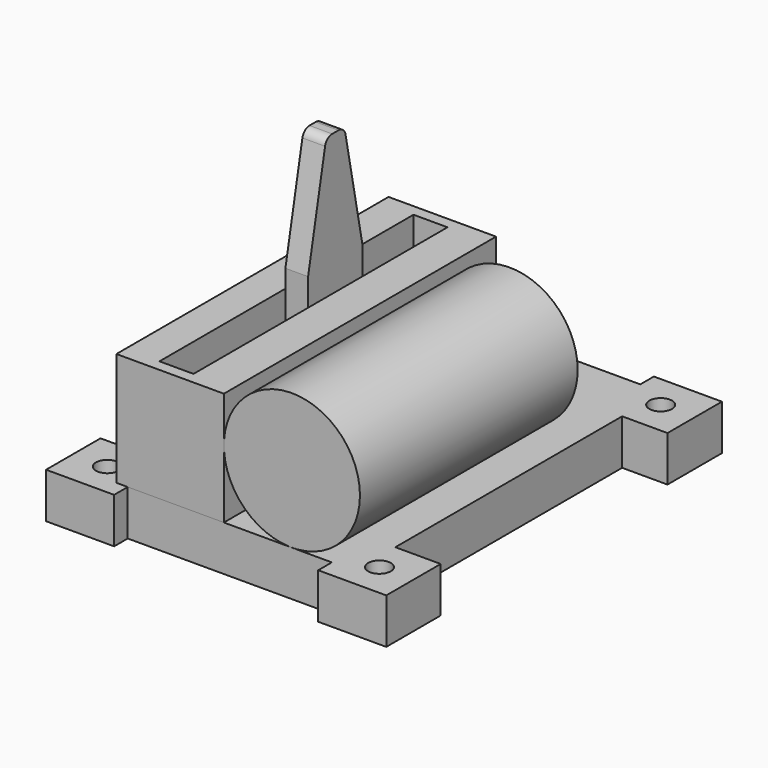
from build123d import *

# Parameters (mm, degrees)
F0_R     = 0.5
F0_W     = 1.5
F0_H     = 14
F1_DEPTH = 2
F3_DEPTH = 5
F4_DEPTH = 2
F5_R     = 3
F6_DEPTH = 12
F2_W     = 1
F2_H     = 3
F7_DEPTH = 11
F8_SIZE2 = 5
F8_SIZE  = 1
F9_SIZE2 = 5
F9_SIZE  = 1
F10_R    = 0.4


with BuildPart() as f1:
    # F0 (on Top) → F1 (new body)
    with BuildSketch(Plane.XY):
        Polygon((-4.7396611795, -5.7187644923), (-4.2396611795, -5.7187644923), (-0.2396611795, -5.7187644923), (-0.2396611795, -5.2187644923), (-1.7396611795, -5.2187644923), (-3.2396611795, -5.2187644923), (-4.7396611795, -5.2187644923), align=None)
        Polygon((-4.2396611795, 12.0312355077), (-7.2396611795, 12.0312355077), (-7.2396611795, 9.0312355077), (-5.2396611795, 9.0312355077), (-5.2396611795, -3.4687644923), (-7.2396611795, -3.4687644923), (-7.2396611795, -6.4687644923), (-4.2396611795, -6.4687644923), (-4.2396611795, -5.7187644923), (-4.7396611795, -5.7187644923), (-4.7396611795, -5.2187644923), (-4.7396611795, 9.2812355077), (-0.2396611795, 9.2812355077), (-0.2396611795, -5.2187644923), (-0.2396611795, -5.7187644923), (4.7603388205, -5.7187644923), (4.7603388205, -6.4687644923), (7.7603388205, -6.4687644923), (7.7603388205, -3.4687644923), (5.7603388205, -3.4687644923), (5.7603388205, 9.0312355077), (7.7603388205, 9.0312355077), (7.7603388205, 12.0312355077), (4.7603388205, 12.0312355077), (4.7603388205, 11.2812355077), (-4.2396611795, 11.2812355077), align=None)
        with Locations((-5.7396611795, -4.9687644923)):
            Circle(F0_R, mode=Mode.SUBTRACT)
        with Locations((6.2603388205, -4.9687644923)):
            Circle(F0_R, mode=Mode.SUBTRACT)
        with Locations((-5.7396611795, 10.5312355077)):
            Circle(F0_R, mode=Mode.SUBTRACT)
        with Locations((6.2603388205, 10.5312355077)):
            Circle(F0_R, mode=Mode.SUBTRACT)
        with Locations((-2.4896611795, 1.7812355077)):
            Rectangle(F0_W, F0_H)
    extrude(amount=F1_DEPTH)



with BuildPart() as f3:
    # F2 (on face) → F3 (new body)
    with BuildSketch(Plane.XY.offset(2)):
        Polygon((-0.2396611795, 9.2812355077), (-4.7396611795, 9.2812355077), (-4.7396611795, -5.2187644923), (-3.2396611795, -5.2187644923), (-3.2396611795, 8.7812355077), (-1.7396611795, 8.7812355077), (-1.7396611795, -5.2187644923), (-0.2396611795, -5.2187644923), align=None)
        Polygon((0, 9.2812355077), (-0.2396611795, 9.2812355077), (-0.2396611795, -5.2187644923), (-1.7396611795, -5.2187644923), (-3.2396611795, -5.2187644923), (-4.7396611795, -5.2187644923), (-4.7396611795, -5.7187644923), (-4.2396611795, -5.7187644923), (0, -5.7187644923), align=None)
    extrude(amount=F3_DEPTH)


with BuildPart() as f1_1:
    add(f1.part)
    # F4 (add): a face of the model
    f4_faces = [f3.part.faces().sort_by_distance(p)[0] for p in [
        (-4.5823511709, 1.7812355077, 2),
    ]]
    extrude(f4_faces, amount=F4_DEPTH)


with BuildPart() as f6:
    # F5 (on face) → F6 (new body)
    with BuildSketch(Plane.XZ.offset(5.7187644923)):
        with Locations((3, 5)):
            Circle(F5_R)
    extrude(amount=-F6_DEPTH)


with BuildPart() as f7:
    # F2 (on face) → F7 (new body)
    with BuildSketch(Plane.XY.offset(2)):
        with Locations((-2.4896611795, 2.910102006)):
            Rectangle(F2_W, F2_H)
    extrude(amount=F7_DEPTH)

    # F8
    f8_edges = [f7.edges().sort_by_distance(p)[0] for p in [
        (-2.489661, 1.410102, 13),
    ]]
    f8_side = f7.faces().sort_by_distance((-2.489661, 2.910102, 13))[0]
    chamfer(f8_edges, length=F8_SIZE, length2=F8_SIZE2, reference=f8_side)

    # F9
    f9_edges = [f7.edges().sort_by_distance(p)[0] for p in [
        (-2.489661, 4.410102, 13),
    ]]
    f9_side = f7.faces().sort_by_distance((-2.489661, 3.410102, 13))[0]
    chamfer(f9_edges, length=F9_SIZE, length2=F9_SIZE2, reference=f9_side)

    # F10
    f10_edges = [f7.edges().sort_by_distance(p)[0] for p in [
        (-2.489661, 3.410102, 13),
        (-2.489661, 2.410102, 13),
    ]]
    fillet(f10_edges, radius=F10_R)


solid = Compound([f3.part, f1_1.part, f6.part, f7.part])
